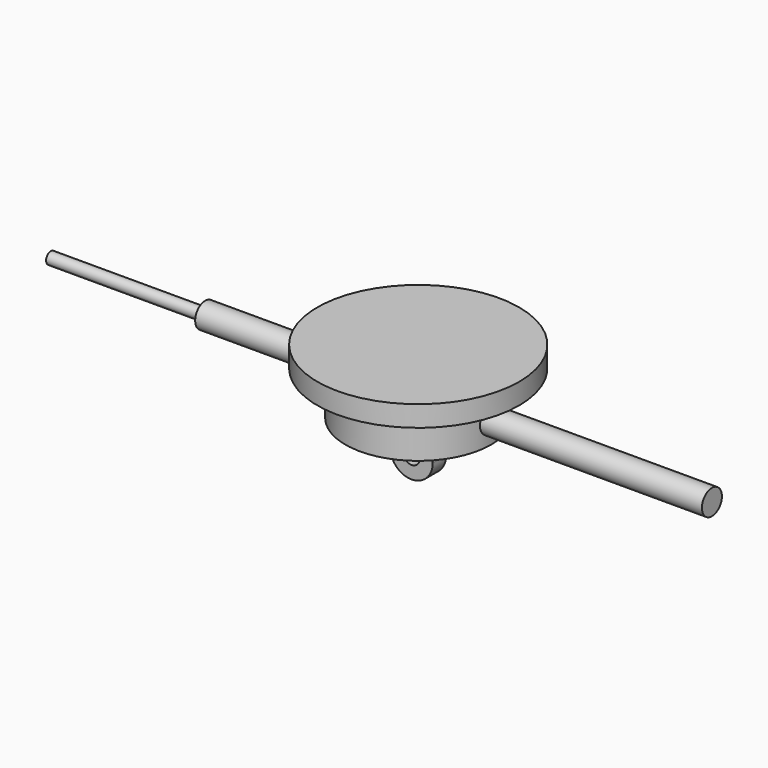
from build123d import *

# Parameters (mm, degrees)
F0_R      = 38.1
F1_DEPTH  = 7.874
F2_R      = 27.4701
F3_DEPTH  = 16.51
F4_R      = 4.7244
F5_DEPTH  = 110.8964
F6_DEPTH  = 80.4672
F7_R      = 2.2352
F8_DEPTH  = 58.293
F9_W      = 16.002
F9_H      = 6.35
F10_DEPTH = 19.177
F11_R     = 8.00099
F13_D     = 6.35


# Not quite as in the source:
# - a fillet or chamfer is up to 0.001 mm smaller than in the source, because OpenCascade refuses the exact size


with BuildPart() as f1:
    # F0 (on Top) → F1 (new body)
    with BuildSketch(Plane.XY):
        Circle(F0_R)
    extrude(amount=F1_DEPTH)

    # F2 (on Top) → F3 (join)
    with BuildSketch(Plane.XY):
        Circle(F2_R)
    extrude(amount=-F3_DEPTH)

    # F4 (on Right) → F5 (join)
    with BuildSketch(Plane.YZ):
        with Locations((0, -8.4328)):
            Circle(F4_R)
    extrude(amount=F5_DEPTH)

    # F4 (on Right) → F6 (join)
    with BuildSketch(Plane.YZ):
        with Locations((0, -8.4328)):
            Circle(F4_R)
    extrude(amount=-F6_DEPTH)

    # F7 (on face) → F8 (join)
    with BuildSketch(Plane(origin=(-80.4672, 0, 0), x_dir=(0, -1, 0), z_dir=(-1, 0, 0))):
        with Locations((0, -8.4328)):
            Circle(F7_R)
    extrude(amount=F8_DEPTH)

    # F9 (on face) → F10 (join)
    with BuildSketch(Plane(origin=(0, 0, -16.51), x_dir=(1, 0, 0), z_dir=(0, 0, -1))):
        Rectangle(F9_W, F9_H)
    extrude(amount=F10_DEPTH)

    # F11 (radius 8.001 in the source; OpenCascade refuses exactly that, so slightly less here)
    f11_edges = [f1.edges().sort_by_distance(p)[0] for p in [
        (8.001, 0, -35.687),
        (-8.001, 0, -35.687),
    ]]
    fillet(f11_edges, radius=F11_R)

    # F13 (through all)
    with Locations(Plane(origin=(0, 3.175, 0), x_dir=(-1, 0, 0), z_dir=(0, 1, 0))):
        with Locations((0, -27.686)):
            Hole(F13_D / 2)


solid = f1.part
